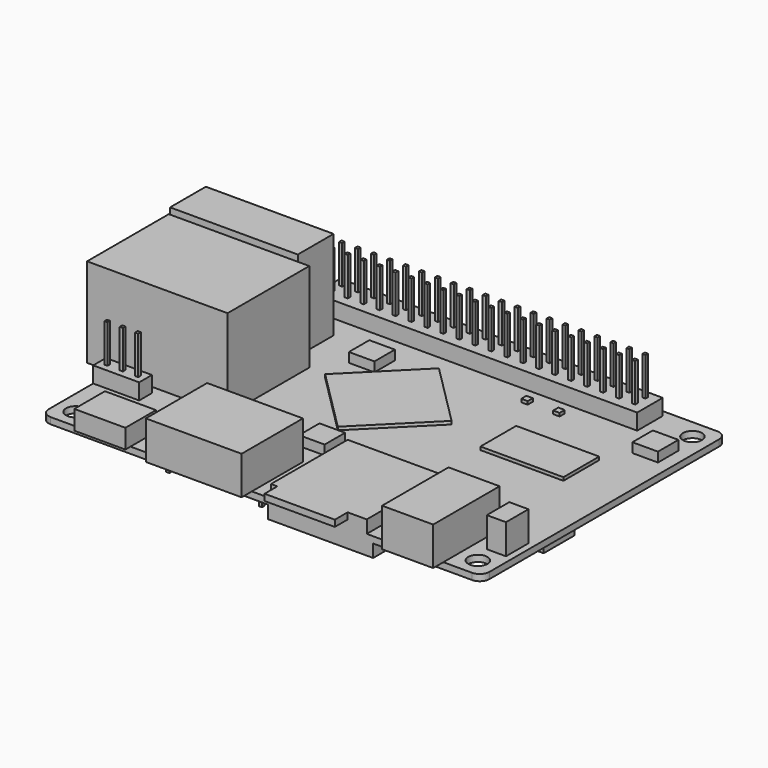
from build123d import *

# Parameters (mm, degrees)
F0_R      = 1.5
F1_DEPTH  = 1
F2_W      = 3
F2_H      = 4.4
F3_DEPTH  = 4.7
F6_W      = 8
F6_H      = 13
F7_DEPTH  = 6
F8_W      = 15
F8_H      = 15
F9_DEPTH  = 2
F10_W     = 11
F10_H     = 1
F11_DEPTH = 2.5
F12_W     = 15
F12_H     = 12
F13_DEPTH = 6
F14_W     = 8
F14_H     = 6
F15_DEPTH = 3
F16_W     = 7.2
F16_H     = 2.5
F17_DEPTH = 2.5
F18_W     = 0.5
F18_H     = 0.5
F19_DEPTH = 6
F20_W     = 22
F20_H     = 16
F21_DEPTH = 14
F22_W     = 20
F22_H     = 7
F23_DEPTH = 14
F24_W     = 50.5
F24_H     = 5
F25_DEPTH = 2.5
F26_W     = 0.5
F26_H     = 0.5
F27_DEPTH = 6
F28_DEPTH = 6
F29_W     = 13
F29_H     = 7
F30_DEPTH = 0.5
F31_W     = 4
F31_H     = 4
F32_DEPTH = 1.5
F33_W     = 1
F33_H     = 1
F34_DEPTH = 0.5
F36_DEPTH = 0.5
F37_DEPTH = 6
F38_W     = 16.5
F38_H     = 6
F39_DEPTH = 2
F40_W     = 4.5
F40_H     = 4.5
F41_DEPTH = 2
F42_W     = 13.5
F42_H     = 7.5
F43_DEPTH = 0.5
F44_W     = 9
F44_H     = 6
F45_DEPTH = 2
F46_W     = 1
F46_H     = 1
F46_W_2   = 0.5
F46_H_2   = 0.5
F47_DEPTH = 3
F48_W     = 3
F48_H     = 3
F48_W_2   = 0.5
F48_H_2   = 2
F48_H_3   = 0.5
F48_W_3   = 1
F48_H_4   = 1
F49_DEPTH = 2


# Not quite as in the source:
# - the program builds the solid bodies; features that only make, move or delete a surface that nothing else refers to are left out


with BuildPart() as f1:
    # F0 (on Top) → F1 (new body)
    with BuildSketch(Plane.XY):
        with BuildLine():
            Line((23.6635117233, 28.4354079459), (-42.3364882767, 28.4354079459))
            ThreePointArc((-42.3364882767, 28.4354079459), (-43.3971484485, 27.9960681177), (-43.8364882767, 26.9354079459))
            Line((-43.8364882767, 26.9354079459), (-43.8364882767, -18.0645920541))
            ThreePointArc((-43.8364882767, -18.0645920541), (-43.3971484485, -19.1252522259), (-42.3364882767, -19.5645920541))
            Line((-42.3364882767, -19.5645920541), (-37.8364882767, -19.5645920541))
            Line((-37.8364882767, -19.5645920541), (19.1635117233, -19.5645920541))
            Line((19.1635117233, -19.5645920541), (23.6635117233, -19.5645920541))
            ThreePointArc((23.6635117233, -19.5645920541), (24.7241718951, -19.1252522259), (25.1635117233, -18.0645920541))
            Line((25.1635117233, -18.0645920541), (25.1635117233, 26.9354079459))
            ThreePointArc((25.1635117233, 26.9354079459), (24.7241718951, 27.9960681177), (23.6635117233, 28.4354079459))
        make_face()
        with Locations((-40.8364882767, -16.5645920541)):
            Circle(F0_R, mode=Mode.SUBTRACT)
        with Locations((22.1635117233, -16.5645920541)):
            Circle(F0_R, mode=Mode.SUBTRACT)
        with Locations((-40.8364882767, 25.4354079459)):
            Circle(F0_R, mode=Mode.SUBTRACT)
        with Locations((22.1635117233, 25.4354079459)):
            Circle(F0_R, mode=Mode.SUBTRACT)
    extrude(amount=F1_DEPTH)

    # F2 (on face) → F3 (join)
    with BuildSketch(Plane.XY.offset(1)):
        with Locations((22.6635117233, -11.3645920541)):
            Rectangle(F2_W, F2_H)
    extrude(amount=F3_DEPTH)

    # F6 (on face) → F7 (join)
    with BuildSketch(Plane.XY.offset(1)):
        with Locations((15.1635117233, -15.0645920541)):
            Rectangle(F6_W, F6_H)
    extrude(amount=F7_DEPTH)

    # F8 (on face) → F9 (join)
    with BuildSketch(Plane.XY.offset(1)):
        with Locations((-0.3364882767, -12.0645920541)):
            Rectangle(F8_W, F8_H)
    extrude(amount=F9_DEPTH)

    # F10 (on face) → F11 (join)
    with BuildSketch(Plane.XZ.offset(19.5645920541)):
        with Locations((-1.3364882767, 2.5)):
            Rectangle(F10_W, F10_H)
    extrude(amount=F11_DEPTH)

    # F12 (on face) → F13 (join)
    with BuildSketch(Plane.XY.offset(1)):
        with Locations((-18.3364882767, -15.5645920541)):
            Rectangle(F12_W, F12_H)
    extrude(amount=F13_DEPTH)

    # F14 (on face) → F15 (join)
    with BuildSketch(Plane.XY.offset(1)):
        with Locations((-33.8364882767, -17.5645920541)):
            Rectangle(F14_W, F14_H)
    extrude(amount=F15_DEPTH)

    # F16 (on face) → F17 (join)
    with BuildSketch(Plane.XY.offset(1)):
        with Locations((-40.2364882767, -8.1145920541)):
            Rectangle(F16_W, F16_H)
    extrude(amount=F17_DEPTH)

    # F18 (on face) → F19 (join)
    with BuildSketch(Plane.XY.offset(3.5)):
        with Locations((-42.6364882767, -8.1145920541)):
            Rectangle(F18_W, F18_H)
        with Locations((-40.2364882767, -8.1145920541)):
            Rectangle(F18_W, F18_H)
        with Locations((-37.8364882767, -8.1145920541)):
            Rectangle(F18_W, F18_H)
    extrude(amount=F19_DEPTH)

    # F20 (on face) → F21 (join)
    with BuildSketch(Plane.XY.offset(1)):
        with Locations((-36.8364882767, 2.4354079459)):
            Rectangle(F20_W, F20_H)
    extrude(amount=F21_DEPTH)

    # F22 (on face) → F23 (join)
    with BuildSketch(Plane.XY.offset(1)):
        with Locations((-38.8364882767, 15.4354079459)):
            Rectangle(F22_W, F22_H)
    extrude(amount=F23_DEPTH)

    # F24 (on face) → F25 (join)
    with BuildSketch(Plane.XY.offset(1)):
        with Locations((-9.3364882767, 24.9354079459)):
            Rectangle(F24_W, F24_H)
    extrude(amount=F25_DEPTH)

    # F26 (on face) → F28 (join)
    with BuildSketch(Plane.XY.offset(3.5)):
        with Locations((-33.3364882767, 26.1854079459)):
            Rectangle(F26_W, F26_H)
        with Locations((-30.8364882767, 26.1854079459)):
            Rectangle(F26_W, F26_H)
        with Locations((-28.3364882767, 26.1854079459)):
            Rectangle(F26_W, F26_H)
        with Locations((-25.8364882767, 26.1854079459)):
            Rectangle(F26_W, F26_H)
        with Locations((-23.3364882767, 26.1854079459)):
            Rectangle(F26_W, F26_H)
        with Locations((-20.8364882767, 26.1854079459)):
            Rectangle(F26_W, F26_H)
        with Locations((-18.3364882767, 26.1854079459)):
            Rectangle(F26_W, F26_H)
        with Locations((-15.8364882767, 26.1854079459)):
            Rectangle(F26_W, F26_H)
        with Locations((-13.3364882767, 26.1854079459)):
            Rectangle(F26_W, F26_H)
        with Locations((-10.8364882767, 26.1854079459)):
            Rectangle(F26_W, F26_H)
        with Locations((-8.3364882767, 26.1854079459)):
            Rectangle(F26_W, F26_H)
        with Locations((-5.8364882767, 26.1854079459)):
            Rectangle(F26_W, F26_H)
        with Locations((-3.3364882767, 26.1854079459)):
            Rectangle(F26_W, F26_H)
        with Locations((-0.8364882767, 26.1854079459)):
            Rectangle(F26_W, F26_H)
        with Locations((1.6635117233, 26.1854079459)):
            Rectangle(F26_W, F26_H)
        with Locations((4.1635117233, 26.1854079459)):
            Rectangle(F26_W, F26_H)
        with Locations((6.6635117233, 26.1854079459)):
            Rectangle(F26_W, F26_H)
        with Locations((9.1635117233, 26.1854079459)):
            Rectangle(F26_W, F26_H)
        with Locations((11.6635117233, 26.1854079459)):
            Rectangle(F26_W, F26_H)
        with Locations((14.1635117233, 26.1854079459)):
            Rectangle(F26_W, F26_H)
        with Locations((14.1588162707, 24.1854134577)):
            Rectangle(F26_W, F26_H)
        with Locations((11.658816397, 24.1846187375)):
            Rectangle(F26_W, F26_H)
        with Locations((9.1588165233, 24.1838240173)):
            Rectangle(F26_W, F26_H)
        with Locations((6.6588166496, 24.1830292971)):
            Rectangle(F26_W, F26_H)
        with Locations((4.1588167759, 24.1822345769)):
            Rectangle(F26_W, F26_H)
        with Locations((1.6588169022, 24.1814398566)):
            Rectangle(F26_W, F26_H)
        with Locations((-0.8411829714, 24.1806451364)):
            Rectangle(F26_W, F26_H)
        with Locations((-3.3411828451, 24.1798504162)):
            Rectangle(F26_W, F26_H)
        with Locations((-5.8411827188, 24.179055696)):
            Rectangle(F26_W, F26_H)
        with Locations((-8.3411825925, 24.1782609758)):
            Rectangle(F26_W, F26_H)
        with Locations((-10.8411824662, 24.1774662556)):
            Rectangle(F26_W, F26_H)
        with Locations((-13.3411823399, 24.1766715354)):
            Rectangle(F26_W, F26_H)
        with Locations((-15.8411822135, 24.1758768152)):
            Rectangle(F26_W, F26_H)
        with Locations((-18.3411820872, 24.1750820949)):
            Rectangle(F26_W, F26_H)
        with Locations((-20.8411819609, 24.1742873747)):
            Rectangle(F26_W, F26_H)
        with Locations((-23.3411818346, 24.1734926545)):
            Rectangle(F26_W, F26_H)
        with Locations((-25.8411817083, 24.1726979343)):
            Rectangle(F26_W, F26_H)
        with Locations((-28.341181582, 24.1719032141)):
            Rectangle(F26_W, F26_H)
        with Locations((-30.8411814556, 24.1711084939)):
            Rectangle(F26_W, F26_H)
        with Locations((-33.3411813293, 24.1703137737)):
            Rectangle(F26_W, F26_H)
    extrude(amount=-F28_DEPTH)

    # F29 (on face) → F30 (join)
    with BuildSketch(Plane.XY.offset(1)):
        with Locations((10.6635117233, 9.9354079459)):
            Rectangle(F29_W, F29_H)
    extrude(amount=F30_DEPTH)

    # F31 (on face) → F32 (join)
    with BuildSketch(Plane.XY.offset(1)):
        with Locations((21.1635117233, 19.4354079459)):
            Rectangle(F31_W, F31_H)
        with Locations((-20.8364882767, 16.4354079459)):
            Rectangle(F31_W, F31_H)
        with Locations((-11.8364882767, -4.5645920541)):
            Rectangle(F31_W, F31_H)
    extrude(amount=F32_DEPTH)

    # F33 (on face) → F34 (join)
    with BuildSketch(Plane.XY.offset(1)):
        with Locations((0.6635117233, 19.9354079459)):
            Rectangle(F33_W, F33_H)
        with Locations((5.6635117233, 19.9354079459)):
            Rectangle(F33_W, F33_H)
    extrude(amount=F34_DEPTH)

    # F35 (on face) → F36 (join)
    with BuildSketch(Plane.XY.offset(1)):
        Polygon((-2.8364882767, 9.5359130093), (-12.7359832133, 19.4354079459), (-22.6354781499, 9.5359130093), (-12.7359832133, -0.3635819273), align=None)
    extrude(amount=F36_DEPTH)

    # F18 (on face) → F37 (join)
    with BuildSketch(Plane.XY.offset(3.5)):
        with Locations((-42.6364882767, -8.1145920541)):
            Rectangle(F18_W, F18_H)
        with Locations((-40.2364882767, -8.1145920541)):
            Rectangle(F18_W, F18_H)
        with Locations((-37.8364882767, -8.1145920541)):
            Rectangle(F18_W, F18_H)
    extrude(amount=-F37_DEPTH)

    # F38 (on face) → F39 (join)
    with BuildSketch(Plane.XY):
        with Locations((-0.0864882767, -16.5645920541)):
            Rectangle(F38_W, F38_H)
    extrude(amount=-F39_DEPTH)

    # F40 (on face) → F41 (join)
    with BuildSketch(Plane.XY):
        with Locations((-1.0864882767, -6.3145920541)):
            Rectangle(F40_W, F40_H)
    extrude(amount=-F41_DEPTH)

    # F42 (on face) → F43 (join)
    with BuildSketch(Plane.XY):
        with Locations((10.4135117233, 8.6854079459)):
            Rectangle(F42_W, F42_H)
    extrude(amount=-F43_DEPTH)

    # F44 (on face) → F45 (join)
    with BuildSketch(Plane.XY):
        with Locations((19.1635117233, -2.5645920541)):
            Rectangle(F44_W, F44_H)
    extrude(amount=-F45_DEPTH)

    # F46 (on face) → F47 (join)
    with BuildSketch(Plane.XY):
        with Locations((-36.3364882767, 11.9354079459)):
            Rectangle(F46_W, F46_H)
        with Locations((-29.3364882767, 11.9354079459)):
            Rectangle(F46_W, F46_H)
        with Locations((-36.3364882767, 18.4354079459)):
            Rectangle(F46_W, F46_H)
        with Locations((-29.3364882767, 18.4354079459)):
            Rectangle(F46_W, F46_H)
        with Locations((-34.3364882767, 9.9354079459)):
            Rectangle(F46_W, F46_H)
        with Locations((-34.3364882767, -0.5645920541)):
            Rectangle(F46_W, F46_H)
        with Locations((-41.0864882767, -4.8145920541)):
            Rectangle(F46_W_2, F46_H_2)
        with Locations((-41.0864882767, -2.3145920541)):
            Rectangle(F46_W_2, F46_H_2)
        with Locations((-30.5864882767, -1.4145920541)):
            Rectangle(F46_W_2, F46_H_2)
        with Locations((-28.3864882767, -2.6145920541)):
            Rectangle(F46_W_2, F46_H_2)
        with Locations((-30.5864882767, 1.2854079459)):
            Rectangle(F46_W_2, F46_H_2)
        with Locations((-28.3864882767, 0.0854079459)):
            Rectangle(F46_W_2, F46_H_2)
        with Locations((-30.5864882767, 3.9854079459)):
            Rectangle(F46_W_2, F46_H_2)
        with Locations((-28.3864882767, 2.7854079459)):
            Rectangle(F46_W_2, F46_H_2)
        with Locations((-30.5864882767, 6.6854079459)):
            Rectangle(F46_W_2, F46_H_2)
        with Locations((-28.3864882767, 5.4854079459)):
            Rectangle(F46_W_2, F46_H_2)
        with Locations((-41.0864882767, 9.1854079459)):
            Rectangle(F46_W_2, F46_H_2)
        with Locations((-41.0864882767, 6.6854079459)):
            Rectangle(F46_W_2, F46_H_2)
    extrude(amount=-F47_DEPTH)

    # F48 (on face) → F49 (join)
    with BuildSketch(Plane.XY):
        with Locations((-37.3364882767, -3.5645920541)):
            Rectangle(F48_W, F48_H)
        with Locations((-37.3364882767, 7.9354079459)):
            Rectangle(F48_W, F48_H)
        with Locations((-25.5864882767, -11.5645920541)):
            Rectangle(F48_W_2, F48_H_2)
        with Locations((-11.0864882767, -11.5645920541)):
            Rectangle(F48_W_2, F48_H_2)
        with Locations((-25.5864882767, -17.3145920541)):
            Rectangle(F48_W_2, F48_H_3)
        with Locations((-11.0864882767, -17.3145920541)):
            Rectangle(F48_W_2, F48_H_3)
        with Locations((11.6635117233, -13.0645920541)):
            Rectangle(F48_W_3, F48_H_4)
        with Locations((13.1635117233, -10.0645920541)):
            Rectangle(F48_W_3, F48_H_4)
        with Locations((16.6635117233, -11.0645920541)):
            Rectangle(F48_W_3, F48_H_4)
    extrude(amount=-F49_DEPTH)


with BuildPart() as f27:
    # F26 (on face) → F27 (new body)
    with BuildSketch(Plane.XY.offset(3.5)):
        with Locations((-33.3364882767, 26.1854079459)):
            Rectangle(F26_W, F26_H)
    extrude(amount=F27_DEPTH)


with BuildPart() as f27b:
    # F26 (on face) → F27, piece 2 (new body)
    with BuildSketch(Plane.XY.offset(3.5)):
        with Locations((-30.8364882767, 26.1854079459)):
            Rectangle(F26_W, F26_H)
    extrude(amount=F27_DEPTH)


with BuildPart() as f27c:
    # F26 (on face) → F27, piece 3 (new body)
    with BuildSketch(Plane.XY.offset(3.5)):
        with Locations((-28.3364882767, 26.1854079459)):
            Rectangle(F26_W, F26_H)
    extrude(amount=F27_DEPTH)


with BuildPart() as f27d:
    # F26 (on face) → F27, piece 4 (new body)
    with BuildSketch(Plane.XY.offset(3.5)):
        with Locations((-25.8364882767, 26.1854079459)):
            Rectangle(F26_W, F26_H)
    extrude(amount=F27_DEPTH)


with BuildPart() as f27e:
    # F26 (on face) → F27, piece 5 (new body)
    with BuildSketch(Plane.XY.offset(3.5)):
        with Locations((-23.3364882767, 26.1854079459)):
            Rectangle(F26_W, F26_H)
    extrude(amount=F27_DEPTH)


with BuildPart() as f27f:
    # F26 (on face) → F27, piece 6 (new body)
    with BuildSketch(Plane.XY.offset(3.5)):
        with Locations((-20.8364882767, 26.1854079459)):
            Rectangle(F26_W, F26_H)
    extrude(amount=F27_DEPTH)


with BuildPart() as f27g:
    # F26 (on face) → F27, piece 7 (new body)
    with BuildSketch(Plane.XY.offset(3.5)):
        with Locations((-18.3364882767, 26.1854079459)):
            Rectangle(F26_W, F26_H)
    extrude(amount=F27_DEPTH)


with BuildPart() as f27h:
    # F26 (on face) → F27, piece 8 (new body)
    with BuildSketch(Plane.XY.offset(3.5)):
        with Locations((-15.8364882767, 26.1854079459)):
            Rectangle(F26_W, F26_H)
    extrude(amount=F27_DEPTH)


with BuildPart() as f27i:
    # F26 (on face) → F27, piece 9 (new body)
    with BuildSketch(Plane.XY.offset(3.5)):
        with Locations((-13.3364882767, 26.1854079459)):
            Rectangle(F26_W, F26_H)
    extrude(amount=F27_DEPTH)


with BuildPart() as f27j:
    # F26 (on face) → F27, piece 10 (new body)
    with BuildSketch(Plane.XY.offset(3.5)):
        with Locations((-10.8364882767, 26.1854079459)):
            Rectangle(F26_W, F26_H)
    extrude(amount=F27_DEPTH)


with BuildPart() as f27k:
    # F26 (on face) → F27, piece 11 (new body)
    with BuildSketch(Plane.XY.offset(3.5)):
        with Locations((-8.3364882767, 26.1854079459)):
            Rectangle(F26_W, F26_H)
    extrude(amount=F27_DEPTH)


with BuildPart() as f27l:
    # F26 (on face) → F27, piece 12 (new body)
    with BuildSketch(Plane.XY.offset(3.5)):
        with Locations((-5.8364882767, 26.1854079459)):
            Rectangle(F26_W, F26_H)
    extrude(amount=F27_DEPTH)


with BuildPart() as f27m:
    # F26 (on face) → F27, piece 13 (new body)
    with BuildSketch(Plane.XY.offset(3.5)):
        with Locations((-3.3364882767, 26.1854079459)):
            Rectangle(F26_W, F26_H)
    extrude(amount=F27_DEPTH)


with BuildPart() as f27n:
    # F26 (on face) → F27, piece 14 (new body)
    with BuildSketch(Plane.XY.offset(3.5)):
        with Locations((-0.8364882767, 26.1854079459)):
            Rectangle(F26_W, F26_H)
    extrude(amount=F27_DEPTH)


with BuildPart() as f27o:
    # F26 (on face) → F27, piece 15 (new body)
    with BuildSketch(Plane.XY.offset(3.5)):
        with Locations((1.6635117233, 26.1854079459)):
            Rectangle(F26_W, F26_H)
    extrude(amount=F27_DEPTH)


with BuildPart() as f27p:
    # F26 (on face) → F27, piece 16 (new body)
    with BuildSketch(Plane.XY.offset(3.5)):
        with Locations((4.1635117233, 26.1854079459)):
            Rectangle(F26_W, F26_H)
    extrude(amount=F27_DEPTH)


with BuildPart() as f27q:
    # F26 (on face) → F27, piece 17 (new body)
    with BuildSketch(Plane.XY.offset(3.5)):
        with Locations((6.6635117233, 26.1854079459)):
            Rectangle(F26_W, F26_H)
    extrude(amount=F27_DEPTH)


with BuildPart() as f27r:
    # F26 (on face) → F27, piece 18 (new body)
    with BuildSketch(Plane.XY.offset(3.5)):
        with Locations((9.1635117233, 26.1854079459)):
            Rectangle(F26_W, F26_H)
    extrude(amount=F27_DEPTH)


with BuildPart() as f27s:
    # F26 (on face) → F27, piece 19 (new body)
    with BuildSketch(Plane.XY.offset(3.5)):
        with Locations((11.6635117233, 26.1854079459)):
            Rectangle(F26_W, F26_H)
    extrude(amount=F27_DEPTH)


with BuildPart() as f27t:
    # F26 (on face) → F27, piece 20 (new body)
    with BuildSketch(Plane.XY.offset(3.5)):
        with Locations((14.1635117233, 26.1854079459)):
            Rectangle(F26_W, F26_H)
    extrude(amount=F27_DEPTH)


with BuildPart() as f27u:
    # F26 (on face) → F27, piece 21 (new body)
    with BuildSketch(Plane.XY.offset(3.5)):
        with Locations((14.1588162707, 24.1854134577)):
            Rectangle(F26_W, F26_H)
    extrude(amount=F27_DEPTH)


with BuildPart() as f27v:
    # F26 (on face) → F27, piece 22 (new body)
    with BuildSketch(Plane.XY.offset(3.5)):
        with Locations((11.658816397, 24.1846187375)):
            Rectangle(F26_W, F26_H)
    extrude(amount=F27_DEPTH)


with BuildPart() as f27w:
    # F26 (on face) → F27, piece 23 (new body)
    with BuildSketch(Plane.XY.offset(3.5)):
        with Locations((9.1588165233, 24.1838240173)):
            Rectangle(F26_W, F26_H)
    extrude(amount=F27_DEPTH)


with BuildPart() as f27x:
    # F26 (on face) → F27, piece 24 (new body)
    with BuildSketch(Plane.XY.offset(3.5)):
        with Locations((6.6588166496, 24.1830292971)):
            Rectangle(F26_W, F26_H)
    extrude(amount=F27_DEPTH)


with BuildPart() as f27y:
    # F26 (on face) → F27, piece 25 (new body)
    with BuildSketch(Plane.XY.offset(3.5)):
        with Locations((4.1588167759, 24.1822345769)):
            Rectangle(F26_W, F26_H)
    extrude(amount=F27_DEPTH)


with BuildPart() as f27z:
    # F26 (on face) → F27, piece 26 (new body)
    with BuildSketch(Plane.XY.offset(3.5)):
        with Locations((1.6588169022, 24.1814398566)):
            Rectangle(F26_W, F26_H)
    extrude(amount=F27_DEPTH)


with BuildPart() as f27ba:
    # F26 (on face) → F27, piece 27 (new body)
    with BuildSketch(Plane.XY.offset(3.5)):
        with Locations((-0.8411829714, 24.1806451364)):
            Rectangle(F26_W, F26_H)
    extrude(amount=F27_DEPTH)


with BuildPart() as f27bb:
    # F26 (on face) → F27, piece 28 (new body)
    with BuildSketch(Plane.XY.offset(3.5)):
        with Locations((-3.3411828451, 24.1798504162)):
            Rectangle(F26_W, F26_H)
    extrude(amount=F27_DEPTH)


with BuildPart() as f27bc:
    # F26 (on face) → F27, piece 29 (new body)
    with BuildSketch(Plane.XY.offset(3.5)):
        with Locations((-5.8411827188, 24.179055696)):
            Rectangle(F26_W, F26_H)
    extrude(amount=F27_DEPTH)


with BuildPart() as f27bd:
    # F26 (on face) → F27, piece 30 (new body)
    with BuildSketch(Plane.XY.offset(3.5)):
        with Locations((-8.3411825925, 24.1782609758)):
            Rectangle(F26_W, F26_H)
    extrude(amount=F27_DEPTH)


with BuildPart() as f27be:
    # F26 (on face) → F27, piece 31 (new body)
    with BuildSketch(Plane.XY.offset(3.5)):
        with Locations((-10.8411824662, 24.1774662556)):
            Rectangle(F26_W, F26_H)
    extrude(amount=F27_DEPTH)


with BuildPart() as f27bf:
    # F26 (on face) → F27, piece 32 (new body)
    with BuildSketch(Plane.XY.offset(3.5)):
        with Locations((-13.3411823399, 24.1766715354)):
            Rectangle(F26_W, F26_H)
    extrude(amount=F27_DEPTH)


with BuildPart() as f27bg:
    # F26 (on face) → F27, piece 33 (new body)
    with BuildSketch(Plane.XY.offset(3.5)):
        with Locations((-15.8411822135, 24.1758768152)):
            Rectangle(F26_W, F26_H)
    extrude(amount=F27_DEPTH)


with BuildPart() as f27bh:
    # F26 (on face) → F27, piece 34 (new body)
    with BuildSketch(Plane.XY.offset(3.5)):
        with Locations((-18.3411820872, 24.1750820949)):
            Rectangle(F26_W, F26_H)
    extrude(amount=F27_DEPTH)


with BuildPart() as f27bi:
    # F26 (on face) → F27, piece 35 (new body)
    with BuildSketch(Plane.XY.offset(3.5)):
        with Locations((-20.8411819609, 24.1742873747)):
            Rectangle(F26_W, F26_H)
    extrude(amount=F27_DEPTH)


with BuildPart() as f27bj:
    # F26 (on face) → F27, piece 36 (new body)
    with BuildSketch(Plane.XY.offset(3.5)):
        with Locations((-23.3411818346, 24.1734926545)):
            Rectangle(F26_W, F26_H)
    extrude(amount=F27_DEPTH)


with BuildPart() as f27bk:
    # F26 (on face) → F27, piece 37 (new body)
    with BuildSketch(Plane.XY.offset(3.5)):
        with Locations((-25.8411817083, 24.1726979343)):
            Rectangle(F26_W, F26_H)
    extrude(amount=F27_DEPTH)


with BuildPart() as f27bl:
    # F26 (on face) → F27, piece 38 (new body)
    with BuildSketch(Plane.XY.offset(3.5)):
        with Locations((-28.341181582, 24.1719032141)):
            Rectangle(F26_W, F26_H)
    extrude(amount=F27_DEPTH)


with BuildPart() as f27bm:
    # F26 (on face) → F27, piece 39 (new body)
    with BuildSketch(Plane.XY.offset(3.5)):
        with Locations((-30.8411814556, 24.1711084939)):
            Rectangle(F26_W, F26_H)
    extrude(amount=F27_DEPTH)


with BuildPart() as f27bn:
    # F26 (on face) → F27, piece 40 (new body)
    with BuildSketch(Plane.XY.offset(3.5)):
        with Locations((-33.3411813293, 24.1703137737)):
            Rectangle(F26_W, F26_H)
    extrude(amount=F27_DEPTH)


solid = Compound([f1.part, f27.part, f27b.part, f27c.part, f27d.part, f27e.part, f27f.part, f27g.part, f27h.part, f27i.part, f27j.part, f27k.part, f27l.part, f27m.part, f27n.part, f27o.part, f27p.part, f27q.part, f27r.part, f27s.part, f27t.part, f27u.part, f27v.part, f27w.part, f27x.part, f27y.part, f27z.part, f27ba.part, f27bb.part, f27bc.part, f27bd.part, f27be.part, f27bf.part, f27bg.part, f27bh.part, f27bi.part, f27bj.part, f27bk.part, f27bl.part, f27bm.part, f27bn.part])
